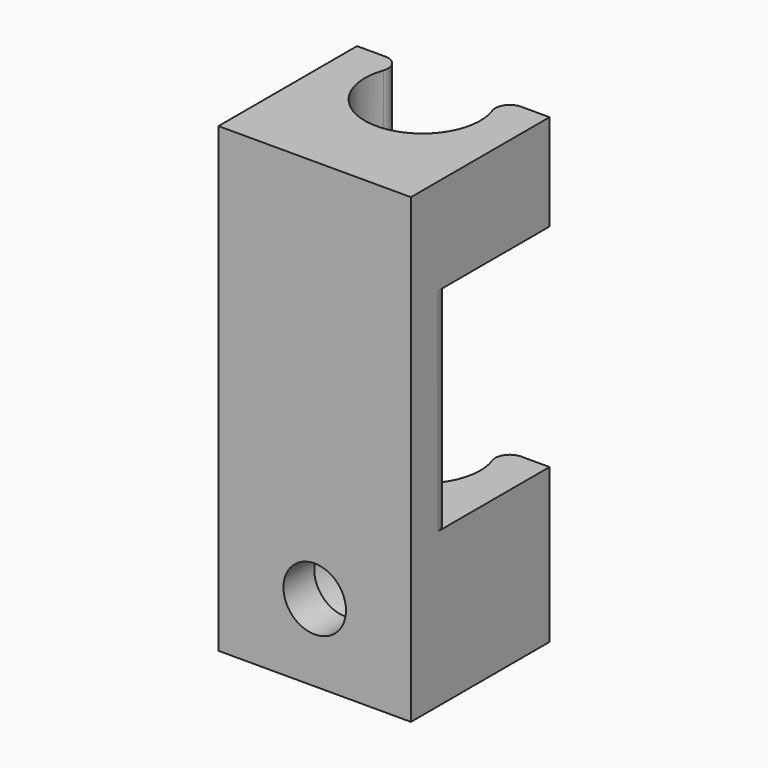
from build123d import *

# Parameters (mm, degrees)
F1_DEPTH  = 25
F2_DEPTH  = 1
F3_DEPTH  = 1
F4_W      = 6
F4_H      = 11
F4_H_2    = 1
F5_DEPTH  = 25
F6_R      = 3
F6_R_2    = 1.625
F7_DEPTH  = 7
F8_DEPTH  = 2
F9_DEPTH  = 1
F10_R     = 0.75
F11_DEPTH = 0.5
F12_R     = 0.75


with BuildPart() as f1:
    # F0 (on Top) → F1 (new body)
    with BuildSketch(Plane.XY):
        with BuildLine():
            Line((0, 9), (0, 0))
            Line((0, 0), (12, 0))
            Line((12, 0), (12, 9))
            Line((12, 9), (8.2360679775, 9))
            ThreePointArc((8.2360679775, 9), (6, 4), (3.7639320225, 9))
            Line((3.7639320225, 9), (0, 9))
        make_face()
    extrude(amount=F1_DEPTH)

    # F2 (cut): a face of the model
    f2_faces = [f1.faces().sort_by_distance(p)[0] for p in [
        (0, 4.5, 12.5),
    ]]
    extrude(f2_faces, amount=-F2_DEPTH, mode=Mode.SUBTRACT)

    # F3 (cut): a face of the model
    f3_faces = [f1.faces().sort_by_distance(p)[0] for p in [
        (12, 4.5, 12.5),
    ]]
    extrude(f3_faces, amount=-F3_DEPTH, mode=Mode.SUBTRACT)

    # F4 (on face) → F5 (cut)
    with BuildSketch(Plane.YZ.offset(11)):
        with Locations((6, 14.5)):
            Rectangle(F4_W, F4_H)
        with Locations((6, 0.5)):
            Rectangle(F4_W, F4_H_2)
    extrude(amount=-F5_DEPTH, mode=Mode.SUBTRACT)

    # F6 (on face) → F7 (cut)
    with BuildSketch(Plane.XZ):
        with Locations((6, 5)):
            Circle(F6_R)
        with Locations((6, 5)):
            Circle(F6_R_2, mode=Mode.SUBTRACT)
        with Locations((6, 5)):
            Circle(F6_R_2)
    extrude(amount=-F7_DEPTH, mode=Mode.SUBTRACT)

    # F6 (on face) → F8 (join)
    with BuildSketch(Plane.XZ):
        with Locations((6, 5)):
            Circle(F6_R)
        with Locations((6, 5)):
            Circle(F6_R_2, mode=Mode.SUBTRACT)
    extrude(amount=-F8_DEPTH)

    # F9 (cut): a face of the model
    f9_faces = [f1.faces().sort_by_distance(p)[0] for p in [
        (6, 1.5, 0),
    ]]
    extrude(f9_faces, amount=-F9_DEPTH, mode=Mode.SUBTRACT)

    # F10
    f10_edges = [f1.edges().sort_by_distance(p)[0] for p in [
        (8.236068, 9, 5),
        (3.763932, 9, 5),
        (3.763932, 9, 22.5),
        (8.236068, 9, 22.5),
    ]]
    fillet(f10_edges, radius=F10_R)

    # F11 (cut): a face of the model
    f11_faces = [f1.faces().sort_by_distance(p)[0] for p in [
        (6, 3, 14.5),
    ]]
    extrude(f11_faces, amount=-F11_DEPTH, mode=Mode.SUBTRACT)

    # F12
    f12_edges = [f1.edges().sort_by_distance(p)[0] for p in [
        (11, 2.5, 14.5),
        (1, 2.5, 14.5),
    ]]
    fillet(f12_edges, radius=F12_R)


solid = f1.part
